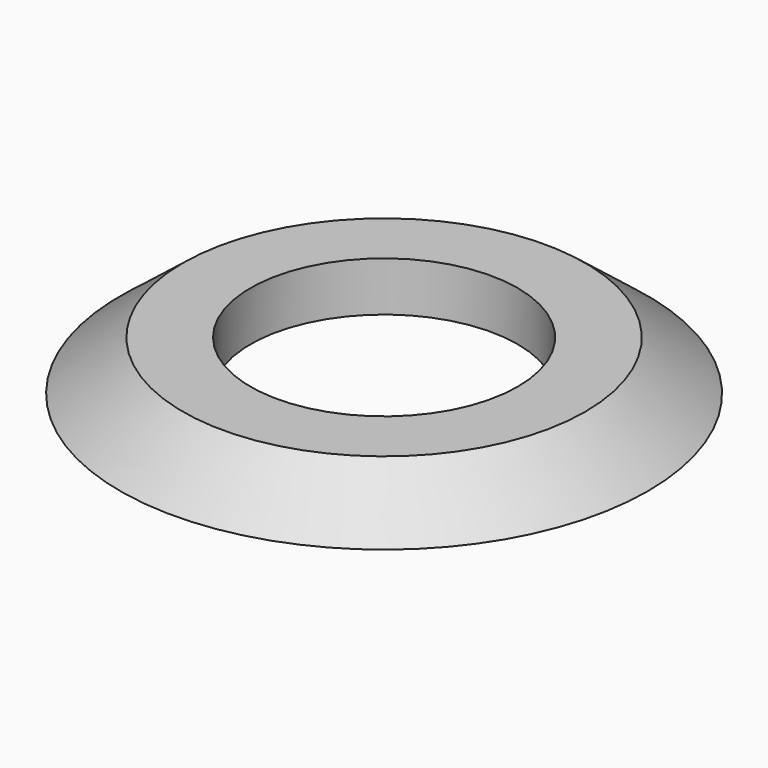
from build123d import *

# Parameters (mm, degrees)
F0_R     = 8
F0_R_2   = 6.05
F0_R_3   = 4.05
F1_DEPTH = 1.5
F2_SIZE2 = 1.49999
F2_SIZE  = 1.89999


# Not quite as in the source:
# - a fillet or chamfer is up to 0.001 mm smaller than in the source, because OpenCascade refuses the exact size


with BuildPart() as f1:
    # F0 (on Top) → F1 (new body)
    with BuildSketch(Plane.XY):
        Circle(F0_R)
        Circle(F0_R_2, mode=Mode.SUBTRACT)
        Circle(F0_R_2)
        Circle(F0_R_3, mode=Mode.SUBTRACT)
    extrude(amount=F1_DEPTH)

    # F2 (size 1.9 and 1.5 in the source; OpenCascade refuses exactly that, so slightly less here)
    f2_edges = [f1.edges().sort_by_distance(p)[0] for p in [
        (-8, 0, 1.5),
    ]]
    f2_side = f1.faces().sort_by_distance((-4.276274, 0, 1.5))[0]
    chamfer(f2_edges, length=F2_SIZE, length2=F2_SIZE2, reference=f2_side)


solid = f1.part
